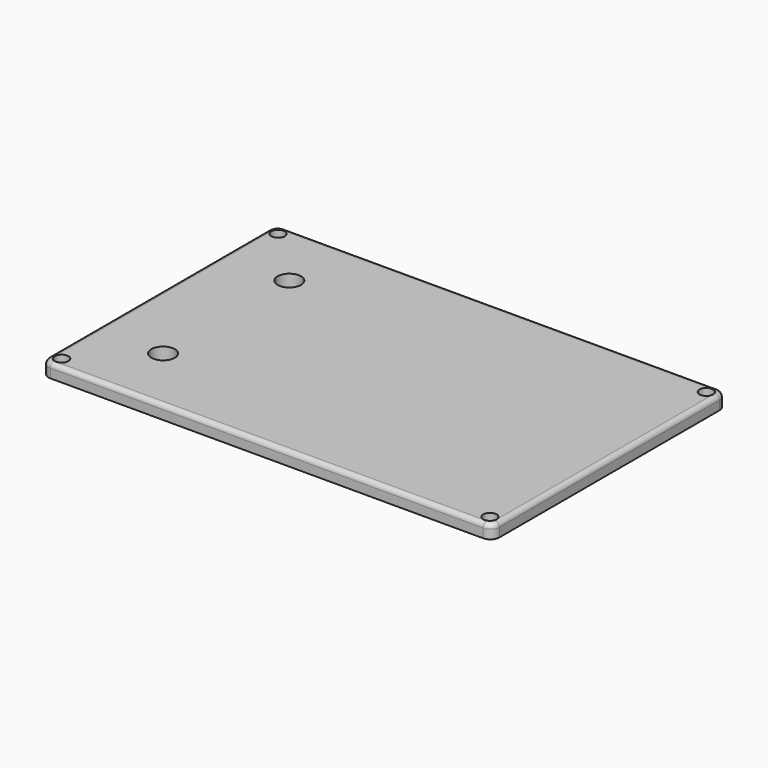
from build123d import *

# Parameters (mm, degrees)
F0_W         = 100
F0_H         = 65
F0_R         = 1.5
F0_R_2       = 2.6
F1_DEPTH     = 3
F2_R         = 0.99999
F3_T1_DEPTH  = 8
F3_T4_ANGLE  = 90
F3_T6_ANGLE  = 90
F3_T8_ANGLE  = 90
F3_T10_ANGLE = 90
F4_W         = 89
F4_H         = 54
F4_R         = 2.6
F5_DEPTH     = 1.5


# Not quite as in the source:
# - a fillet or chamfer that OpenCascade refuses, or shapes differently, is made with other operations: its cross-section is extruded or revolved along the edge and cut away or added
# - a fillet or chamfer is up to 0.001 mm smaller than in the source, because OpenCascade refuses the exact size


with BuildPart() as f1:
    # F0 (on Top) → F1 (new body)
    with BuildSketch(Plane.XY):
        with Locations((4.8531983048, -13.4167700263)):
            Rectangle(F0_W, F0_H)
        with Locations((-42.6468016952, -43.4167700263)):
            Circle(F0_R, mode=Mode.SUBTRACT)
        with Locations((-30.1468016952, -30.9167700263)):
            Circle(F0_R_2, mode=Mode.SUBTRACT)
        with Locations((52.3531983048, -43.4167700263)):
            Circle(F0_R, mode=Mode.SUBTRACT)
        with Locations((-30.1468016952, 4.0832299737)):
            Circle(F0_R_2, mode=Mode.SUBTRACT)
        with Locations((-42.6468016952, 16.5832299737)):
            Circle(F0_R, mode=Mode.SUBTRACT)
        with Locations((52.3531983048, 16.5832299737)):
            Circle(F0_R, mode=Mode.SUBTRACT)
    extrude(amount=F1_DEPTH)

    # F2 (radius 1 in the source; OpenCascade refuses exactly that, so slightly less here)
    f2_edges = [f1.edges().sort_by_distance(p)[0] for p in [
        (-45.146802, -13.41677, 3),
        (4.853198, 19.08323, 3),
        (54.853198, -13.41677, 3),
        (4.853198, -45.91677, 3),
    ]]
    fillet(f2_edges, radius=F2_R)

    # F3: fillet of radius 2 on 4 edges, made by hand

    # F3_s2 → F3_t1 (cut)
    with BuildSketch(Plane.XY.offset(-5)):
        with BuildLine():
            ThreePointArc((-43.1468016952, -45.9167700263), (-44.5610152576, -45.3309835887), (-45.1468016952, -43.9167700263))
            Line((-45.1468016952, -43.9167700263), (-45.1468016952, -45.9167700263))
            Line((-45.1468016952, -45.9167700263), (-43.1468016952, -45.9167700263))
        make_face()
        with BuildLine():
            ThreePointArc((-43.1468016952, 19.0832299737), (-44.5610152576, 18.4974435361), (-45.1468016952, 17.0832299737))
            Line((-45.1468016952, 17.0832299737), (-45.1468016952, 19.0832299737))
            Line((-45.1468016952, 19.0832299737), (-43.1468016952, 19.0832299737))
        make_face()
        with BuildLine():
            ThreePointArc((54.8531983048, 17.0832299737), (54.2674118671, 18.4974435361), (52.8531983048, 19.0832299737))
            Line((52.8531983048, 19.0832299737), (54.8531983048, 19.0832299737))
            Line((54.8531983048, 19.0832299737), (54.8531983048, 17.0832299737))
        make_face()
        with BuildLine():
            ThreePointArc((54.8531983048, -43.9167700263), (54.2674118671, -45.3309835887), (52.8531983048, -45.9167700263))
            Line((52.8531983048, -45.9167700263), (54.8531983048, -45.9167700263))
            Line((54.8531983048, -45.9167700263), (54.8531983048, -43.9167700263))
        make_face()
    extrude(amount=F3_T1_DEPTH, mode=Mode.SUBTRACT)

    # F3_s3 → F3_t4 (revolve, cut)
    with BuildSketch(Plane.YZ.offset(52.8531983048)):
        with BuildLine():
            ThreePointArc((-44.9167800263, 3), (-45.6238797364, 2.7071097101), (-45.9167700263, 2.00001))
            Line((-45.9167700263, 2.00001), (-45.9167700263, 3))
            Line((-45.9167700263, 3), (-44.9167800263, 3))
        make_face()
    revolve(axis=Axis((52.8531983048, -43.9167700263, 3), (0, 0, 1)), revolution_arc=F3_T4_ANGLE, mode=Mode.SUBTRACT)

    # F3_s5 → F3_t6 (revolve, cut)
    with BuildSketch(Plane.XZ.offset(-17.0832299737)):
        with BuildLine():
            ThreePointArc((53.8532083048, 3), (54.5603080149, 2.7071097101), (54.8531983048, 2.00001))
            Line((54.8531983048, 2.00001), (54.8531983048, 3))
            Line((54.8531983048, 3), (53.8532083048, 3))
        make_face()
    revolve(axis=Axis((52.8531983048, 17.0832299737, 3), (0, 0, 1)), revolution_arc=F3_T6_ANGLE, mode=Mode.SUBTRACT)

    # F3_s7 → F3_t8 (revolve, cut)
    with BuildSketch(Plane.YZ.offset(-43.1468016952)):
        with BuildLine():
            ThreePointArc((18.0832399737, 3), (18.7903396838, 2.7071097101), (19.0832299737, 2.00001))
            Line((19.0832299737, 2.00001), (19.0832299737, 3))
            Line((19.0832299737, 3), (18.0832399737, 3))
        make_face()
    revolve(axis=Axis((-43.1468016952, 17.0832299737, 3), (0, 0, 1)), revolution_arc=F3_T8_ANGLE, mode=Mode.SUBTRACT)

    # F3_s9 → F3_t10 (revolve, cut)
    with BuildSketch(Plane.XZ.offset(43.9167700263)):
        with BuildLine():
            ThreePointArc((-44.1468116952, 3), (-44.8539114053, 2.7071097101), (-45.1468016952, 2.00001))
            Line((-45.1468016952, 2.00001), (-45.1468016952, 3))
            Line((-45.1468016952, 3), (-44.1468116952, 3))
        make_face()
    revolve(axis=Axis((-43.1468016952, -43.9167700263, 3), (0, 0, 1)), revolution_arc=F3_T10_ANGLE, mode=Mode.SUBTRACT)

    # F4 (on face) → F5 (join)
    with BuildSketch(Plane(origin=(0, 0, 0), x_dir=(1, 0, 0), z_dir=(0, 0, -1))):
        with Locations((4.8531983048, 13.4167700263)):
            Rectangle(F4_W, F4_H)
        with Locations((-30.1468016952, -4.0832299737)):
            Circle(F4_R, mode=Mode.SUBTRACT)
        with Locations((-30.1468016952, 30.9167700263)):
            Circle(F4_R, mode=Mode.SUBTRACT)
    extrude(amount=F5_DEPTH)


solid = f1.part
